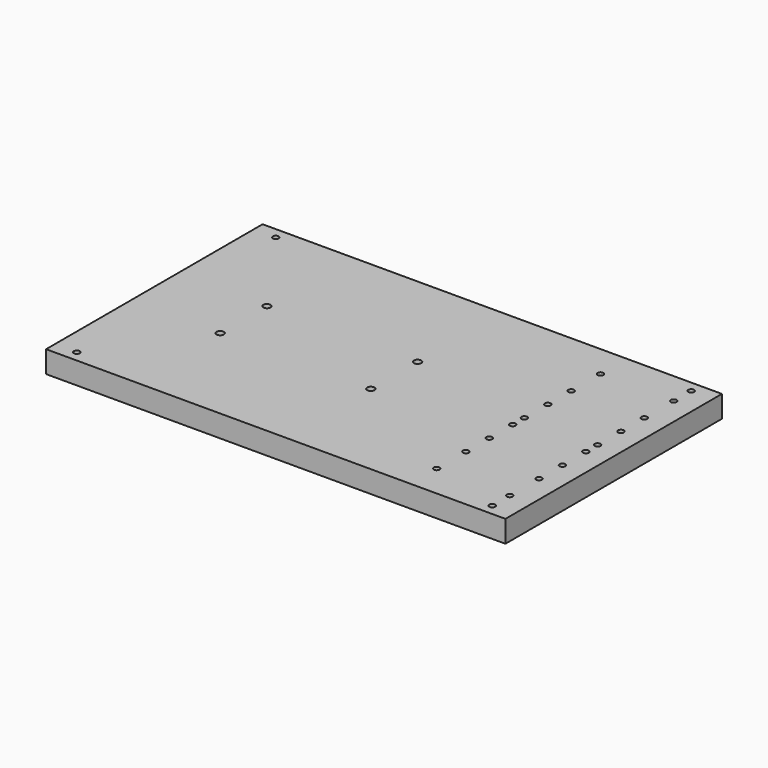
from build123d import *

# Parameters (mm, degrees)
F0_W     = 314
F0_H     = 185
F0_R     = 4
F0_R_2   = 2.5
F0_R_3   = 2
F1_DEPTH = 15
F2_DEPTH = 6


# Not quite as in the source:
# - a feature names something its author has since deleted; it is built from what else it names


with BuildPart() as f1:
    # F0 (on Top) → F1 (new body)
    with BuildSketch(Plane.XY):
        with Locations((-13, 0)):
            Rectangle(F0_W, F0_H)
        with Locations((-155, -85)):
            Circle(F0_R, mode=Mode.SUBTRACT)
        with Locations((-109, -20)):
            Circle(F0_R_2, mode=Mode.SUBTRACT)
        with Locations((79, -70)):
            Circle(F0_R, mode=Mode.SUBTRACT)
        with Locations((129, -85)):
            Circle(F0_R, mode=Mode.SUBTRACT)
        with Locations((129, -70)):
            Circle(F0_R, mode=Mode.SUBTRACT)
        with Locations((-6, -20)):
            Circle(F0_R_2, mode=Mode.SUBTRACT)
        with Locations((79, -45)):
            Circle(F0_R, mode=Mode.SUBTRACT)
        with Locations((79, -25)):
            Circle(F0_R, mode=Mode.SUBTRACT)
        with Locations((129, -45)):
            Circle(F0_R, mode=Mode.SUBTRACT)
        with Locations((129, -25)):
            Circle(F0_R, mode=Mode.SUBTRACT)
        with Locations((79, -5)):
            Circle(F0_R, mode=Mode.SUBTRACT)
        with Locations((129, -5)):
            Circle(F0_R, mode=Mode.SUBTRACT)
        with Locations((-109, 20)):
            Circle(F0_R_2, mode=Mode.SUBTRACT)
        with Locations((-155, 85)):
            Circle(F0_R, mode=Mode.SUBTRACT)
        with Locations((-6, 20)):
            Circle(F0_R_2, mode=Mode.SUBTRACT)
        with Locations((79, 5)):
            Circle(F0_R, mode=Mode.SUBTRACT)
        with Locations((129, 5)):
            Circle(F0_R, mode=Mode.SUBTRACT)
        with Locations((79, 25)):
            Circle(F0_R, mode=Mode.SUBTRACT)
        with Locations((79, 45)):
            Circle(F0_R, mode=Mode.SUBTRACT)
        with Locations((129, 25)):
            Circle(F0_R, mode=Mode.SUBTRACT)
        with Locations((129, 45)):
            Circle(F0_R, mode=Mode.SUBTRACT)
        with Locations((79, 70)):
            Circle(F0_R, mode=Mode.SUBTRACT)
        with Locations((129, 70)):
            Circle(F0_R, mode=Mode.SUBTRACT)
        with Locations((129, 85)):
            Circle(F0_R, mode=Mode.SUBTRACT)
        with Locations((79, 25)):
            Circle(F0_R)
        with Locations((79, 25)):
            Circle(F0_R_3, mode=Mode.SUBTRACT)
        with Locations((79, -70)):
            Circle(F0_R)
        with Locations((79, -70)):
            Circle(F0_R_3, mode=Mode.SUBTRACT)
        with Locations((129, -70)):
            Circle(F0_R)
        with Locations((129, -70)):
            Circle(F0_R_3, mode=Mode.SUBTRACT)
        with Locations((129, -85)):
            Circle(F0_R)
        with Locations((129, -85)):
            Circle(F0_R_3, mode=Mode.SUBTRACT)
        with Locations((129, 85)):
            Circle(F0_R)
        with Locations((129, 85)):
            Circle(F0_R_3, mode=Mode.SUBTRACT)
        with Locations((129, 70)):
            Circle(F0_R)
        with Locations((129, 70)):
            Circle(F0_R_3, mode=Mode.SUBTRACT)
        with Locations((129, 25)):
            Circle(F0_R)
        with Locations((129, 25)):
            Circle(F0_R_3, mode=Mode.SUBTRACT)
        with Locations((79, 70)):
            Circle(F0_R)
        with Locations((79, 70)):
            Circle(F0_R_3, mode=Mode.SUBTRACT)
        with Locations((-155, 85)):
            Circle(F0_R)
        with Locations((-155, 85)):
            Circle(F0_R_3, mode=Mode.SUBTRACT)
        with Locations((-155, -85)):
            Circle(F0_R)
        with Locations((-155, -85)):
            Circle(F0_R_3, mode=Mode.SUBTRACT)
        with Locations((79, 45)):
            Circle(F0_R)
        with Locations((79, 45)):
            Circle(F0_R_3, mode=Mode.SUBTRACT)
        with Locations((79, 5)):
            Circle(F0_R)
        with Locations((79, 5)):
            Circle(F0_R_3, mode=Mode.SUBTRACT)
        with Locations((79, -5)):
            Circle(F0_R)
        with Locations((79, -5)):
            Circle(F0_R_3, mode=Mode.SUBTRACT)
        with Locations((79, -25)):
            Circle(F0_R)
        with Locations((79, -25)):
            Circle(F0_R_3, mode=Mode.SUBTRACT)
        with Locations((79, -45)):
            Circle(F0_R)
        with Locations((79, -45)):
            Circle(F0_R_3, mode=Mode.SUBTRACT)
        with Locations((129, -45)):
            Circle(F0_R)
        with Locations((129, -45)):
            Circle(F0_R_3, mode=Mode.SUBTRACT)
        with Locations((129, -25)):
            Circle(F0_R)
        with Locations((129, -25)):
            Circle(F0_R_3, mode=Mode.SUBTRACT)
        with Locations((129, -5)):
            Circle(F0_R)
        with Locations((129, -5)):
            Circle(F0_R_3, mode=Mode.SUBTRACT)
        with Locations((129, 5)):
            Circle(F0_R)
        with Locations((129, 5)):
            Circle(F0_R_3, mode=Mode.SUBTRACT)
        with Locations((129, 45)):
            Circle(F0_R)
        with Locations((129, 45)):
            Circle(F0_R_3, mode=Mode.SUBTRACT)
    extrude(amount=F1_DEPTH)

    # F0 (on Top) → F2 (cut)
    with BuildSketch(Plane.XY):
        with Locations((79, 25)):
            Circle(F0_R)
        with Locations((79, 25)):
            Circle(F0_R_3, mode=Mode.SUBTRACT)
        with Locations((129, 25)):
            Circle(F0_R)
        with Locations((129, 25)):
            Circle(F0_R_3, mode=Mode.SUBTRACT)
        with Locations((129, 70)):
            Circle(F0_R)
        with Locations((129, 70)):
            Circle(F0_R_3, mode=Mode.SUBTRACT)
        with Locations((79, 70)):
            Circle(F0_R)
        with Locations((79, 70)):
            Circle(F0_R_3, mode=Mode.SUBTRACT)
        with Locations((79, -70)):
            Circle(F0_R)
        with Locations((79, -70)):
            Circle(F0_R_3, mode=Mode.SUBTRACT)
        with Locations((129, -70)):
            Circle(F0_R)
        with Locations((129, -70)):
            Circle(F0_R_3, mode=Mode.SUBTRACT)
        with Locations((79, 45)):
            Circle(F0_R)
        with Locations((79, 45)):
            Circle(F0_R_3, mode=Mode.SUBTRACT)
        with Locations((129, 45)):
            Circle(F0_R)
        with Locations((129, 45)):
            Circle(F0_R_3, mode=Mode.SUBTRACT)
        with Locations((129, 5)):
            Circle(F0_R)
        with Locations((129, 5)):
            Circle(F0_R_3, mode=Mode.SUBTRACT)
        with Locations((129, -5)):
            Circle(F0_R)
        with Locations((129, -5)):
            Circle(F0_R_3, mode=Mode.SUBTRACT)
        with Locations((129, -25)):
            Circle(F0_R)
        with Locations((129, -25)):
            Circle(F0_R_3, mode=Mode.SUBTRACT)
        with Locations((129, -45)):
            Circle(F0_R)
        with Locations((129, -45)):
            Circle(F0_R_3, mode=Mode.SUBTRACT)
        with Locations((79, -45)):
            Circle(F0_R)
        with Locations((79, -45)):
            Circle(F0_R_3, mode=Mode.SUBTRACT)
        with Locations((79, -25)):
            Circle(F0_R)
        with Locations((79, -25)):
            Circle(F0_R_3, mode=Mode.SUBTRACT)
        with Locations((79, -5)):
            Circle(F0_R)
        with Locations((79, -5)):
            Circle(F0_R_3, mode=Mode.SUBTRACT)
        with Locations((79, 5)):
            Circle(F0_R)
        with Locations((79, 5)):
            Circle(F0_R_3, mode=Mode.SUBTRACT)
    extrude(amount=F2_DEPTH, mode=Mode.SUBTRACT)


solid = f1.part
